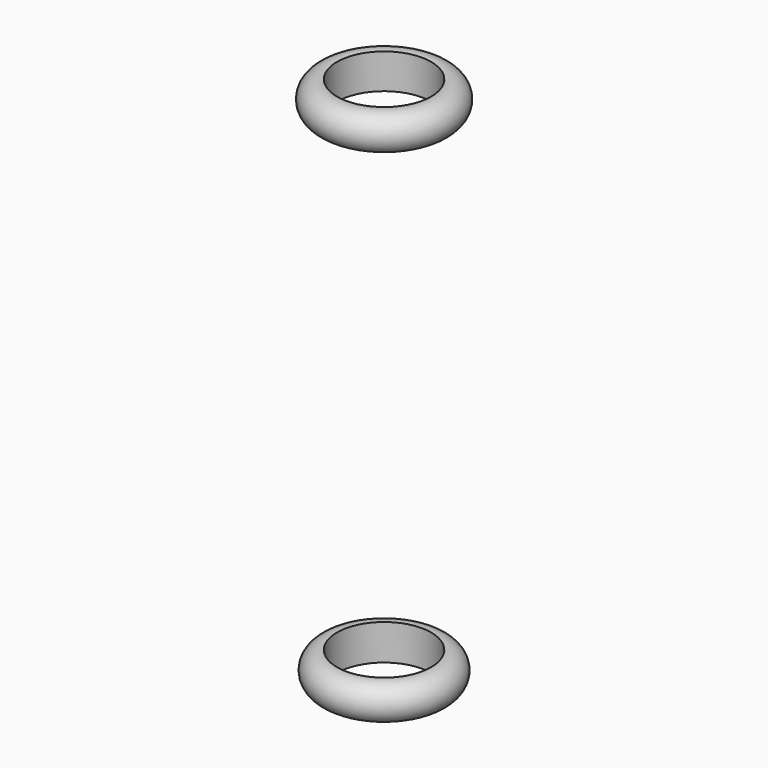
from build123d import *


# Not quite as in the source:
# - the program builds the solid bodies; features that only make, move or delete a surface that nothing else refers to are left out


with BuildPart() as f2:
    # F0 (on Front) → F2 (revolve)
    with BuildSketch(Plane.XZ):
        with BuildLine():
            ThreePointArc((26.67, 55.0053439078), (39.0087231115, 64.9289906974), (26.67, 74.8526374869))
            Line((26.67, 74.8526374869), (26.67, 55.0053439078))
        make_face()
    revolve(axis=Axis((0, 0, 0), (0, 0, -1)))


with BuildPart() as f2b:
    # F0 (on Front) → F2, piece 2 (revolve)
    with BuildSketch(Plane.XZ):
        with BuildLine():
            ThreePointArc((26.67, -229.9473625131), (37.836382144, -219.8373281422), (26.67, -209.7272937714))
            Line((26.67, -209.7272937714), (26.67, -229.9473625131))
        make_face()
    revolve(axis=Axis((0, 0, 0), (0, 0, -1)))


solid = Compound([f2.part, f2b.part])
